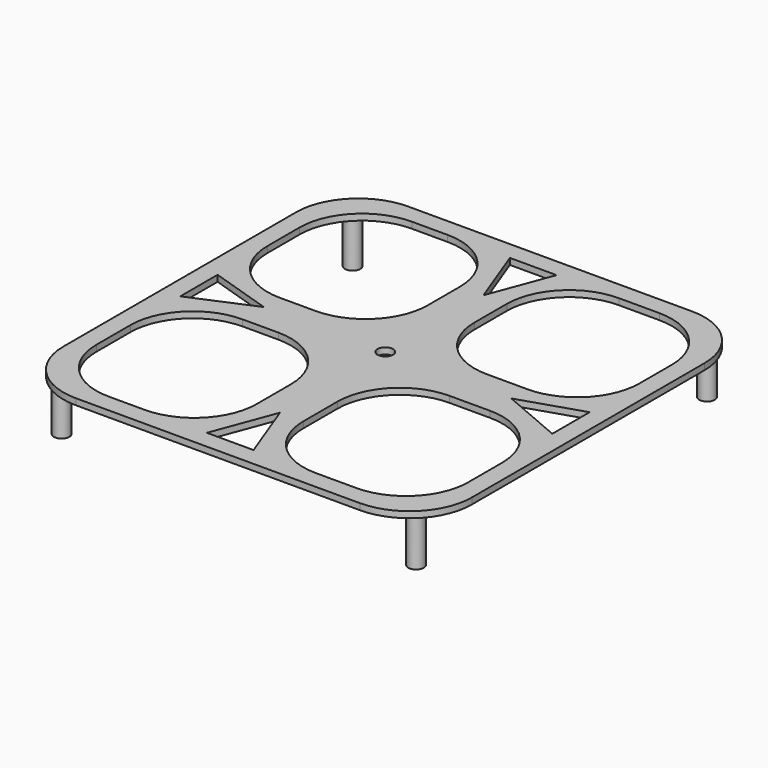
from build123d import *

# Parameters (mm, degrees)
F0_R     = 6.35
F1_DEPTH = 5.08
F2_R     = 6.35
F3_DEPTH = 38.1


# Not quite as in the source:
# - a feature names something its author has since deleted; it is built from what else it names


with BuildPart() as f1:
    # F0 (on Top) → F1 (new body)
    with BuildSketch(Plane.XY):
        with BuildLine():
            ThreePointArc((-164.7597998381, -122.2357259512), (-149.8808243223, -158.1567504355), (-113.9597998381, -173.0357259512))
            Line((-113.9597998381, -173.0357259512), (117.6952974319, -173.0357259512))
            ThreePointArc((117.6952974319, -173.0357259512), (153.6163219162, -158.1567504355), (168.4952974319, -122.2357259512))
            Line((168.4952974319, -122.2357259512), (168.4952974319, 114.9484769821))
            ThreePointArc((168.4952974319, 114.9484769821), (153.6163219162, 150.8695014664), (117.6952974319, 165.7484769821))
            Line((117.6952974319, 165.7484769821), (-113.9597998381, 165.7484769821))
            ThreePointArc((-113.9597998381, 165.7484769821), (-149.8808243223, 150.8695014664), (-164.7597998381, 114.9484769821))
            Line((-164.7597998381, 114.9484769821), (-164.7597998381, -122.2357259512))
        make_face()
        with BuildLine():
            ThreePointArc((-69.85, -21.7389110476), (-33.9289755157, -36.6178865633), (-19.05, -72.5389110476))
            Line((-19.05, -72.5389110476), (-19.05, -107.3567504355))
            ThreePointArc((-19.05, -107.3567504355), (-33.9289755157, -143.2777749197), (-69.85, -158.1567504355))
            Line((-69.85, -158.1567504355), (-99.0808243223, -158.1567504355))
            ThreePointArc((-99.0808243223, -158.1567504355), (-135.0018488066, -143.2777749197), (-149.8808243223, -107.3567504355))
            Line((-149.8808243223, -107.3567504355), (-149.8808243223, -72.5389110476))
            ThreePointArc((-149.8808243223, -72.5389110476), (-135.0018488066, -36.6178865633), (-99.0808243223, -21.7389110476))
            Line((-99.0808243223, -21.7389110476), (-69.85, -21.7389110476))
        make_face(mode=Mode.SUBTRACT)
        Polygon((-19.05, -158.1567504355), (0, -107.3567504355), (19.05, -158.1567504355), align=None, mode=Mode.SUBTRACT)
        with BuildLine():
            Line((69.85, -21.7389110476), (102.8163219162, -21.7389110476))
            ThreePointArc((102.8163219162, -21.7389110476), (138.7373464005, -36.6178865633), (153.6163219162, -72.5389110476))
            Line((153.6163219162, -72.5389110476), (153.6163219162, -107.3567504355))
            ThreePointArc((153.6163219162, -107.3567504355), (138.7373464005, -143.2777749197), (102.8163219162, -158.1567504355))
            Line((102.8163219162, -158.1567504355), (69.85, -158.1567504355))
            ThreePointArc((69.85, -158.1567504355), (33.9289755157, -143.2777749197), (19.05, -107.3567504355))
            Line((19.05, -107.3567504355), (19.05, -72.5389110476))
            ThreePointArc((19.05, -72.5389110476), (33.9289755157, -36.6178865633), (69.85, -21.7389110476))
        make_face(mode=Mode.SUBTRACT)
        Polygon((-149.8808243223, -21.7389110476), (-149.8808243223, 16.3610889524), (-99.0808243223, 0), align=None, mode=Mode.SUBTRACT)
        Circle(F0_R, mode=Mode.SUBTRACT)
        with BuildLine():
            ThreePointArc((-69.85, 150.8695014664), (-33.9289755157, 135.9905259507), (-19.05, 100.0695014664))
            Line((-19.05, 100.0695014664), (-19.05, 67.1610889524))
            ThreePointArc((-19.05, 67.1610889524), (-33.9289755157, 31.2400644681), (-69.85, 16.3610889524))
            Line((-69.85, 16.3610889524), (-99.0808243223, 16.3610889524))
            ThreePointArc((-99.0808243223, 16.3610889524), (-135.0018488066, 31.2400644681), (-149.8808243223, 67.1610889524))
            Line((-149.8808243223, 67.1610889524), (-149.8808243223, 100.0695014664))
            ThreePointArc((-149.8808243223, 100.0695014664), (-135.0018488066, 135.9905259507), (-99.0808243223, 150.8695014664))
            Line((-99.0808243223, 150.8695014664), (-69.85, 150.8695014664))
        make_face(mode=Mode.SUBTRACT)
        Polygon((19.05, 150.8695014664), (0, 100.0695014664), (-19.05, 150.8695014664), align=None, mode=Mode.SUBTRACT)
        Polygon((153.6163219162, -21.7389110476), (102.8163219162, 0), (153.6163219162, 16.3610889524), align=None, mode=Mode.SUBTRACT)
        with BuildLine():
            ThreePointArc((153.6163219162, 67.1610889524), (138.7373464005, 31.2400644681), (102.8163219162, 16.3610889524))
            Line((102.8163219162, 16.3610889524), (69.85, 16.3610889524))
            ThreePointArc((69.85, 16.3610889524), (33.9289755157, 31.2400644681), (19.05, 67.1610889524))
            Line((19.05, 67.1610889524), (19.05, 100.0695014664))
            ThreePointArc((19.05, 100.0695014664), (33.9289755157, 135.9905259507), (69.85, 150.8695014664))
            Line((69.85, 150.8695014664), (102.8163219162, 150.8695014664))
            ThreePointArc((102.8163219162, 150.8695014664), (138.7373464005, 135.9905259507), (153.6163219162, 100.0695014664))
            Line((153.6163219162, 100.0695014664), (153.6163219162, 67.1610889524))
        make_face(mode=Mode.SUBTRACT)
    extrude(amount=F1_DEPTH)

    # F2 (on Top) → F3 (join)
    with BuildSketch(Plane.XY):
        with Locations((-142.0295983553, -152.4900346994)):
            Circle(F2_R)
        with Locations((-142.0295983553, 144.2388147116)):
            Circle(F2_R)
        with Locations((147.0908075571, 144.2388147116)):
            Circle(F2_R)
        with Locations((147.0908075571, -152.4900346994)):
            Circle(F2_R)
    extrude(amount=-F3_DEPTH)


solid = f1.part
